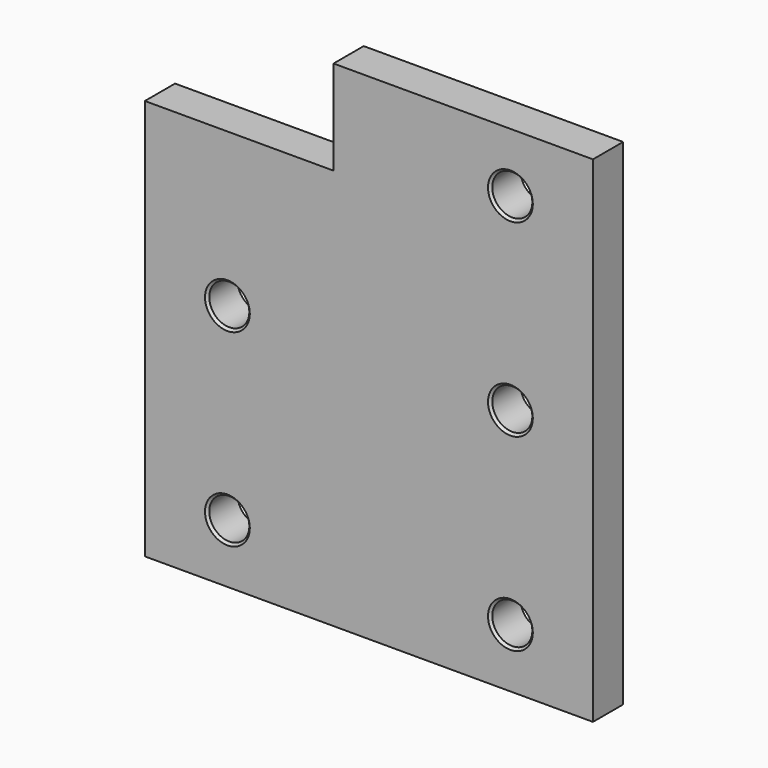
from build123d import *

# Parameters (mm, degrees)
F0_W     = 95
F0_H     = 105
F0_R     = 4.25
F1_DEPTH = 8
F2_SIZE  = 0.5
F3_W     = 50
F3_H     = 55.8646805584
F4_DEPTH = 25


with BuildPart() as f1:
    # F0 (on Front) → F1 (new body)
    with BuildSketch(Plane.XZ):
        with Locations((2.5, 0)):
            Rectangle(F0_W, F0_H)
        with Locations((-27.5, -40)):
            Circle(F0_R, mode=Mode.SUBTRACT)
        with Locations((32.5, -40)):
            Circle(F0_R, mode=Mode.SUBTRACT)
        with Locations((-27.5, 0)):
            Circle(F0_R, mode=Mode.SUBTRACT)
        with Locations((32.5, 0)):
            Circle(F0_R, mode=Mode.SUBTRACT)
        with Locations((32.5, 40)):
            Circle(F0_R, mode=Mode.SUBTRACT)
    extrude(amount=F1_DEPTH)

    # F2
    f2_edges = [f1.edges().sort_by_distance(p)[0] for p in [
        (28.25, -8, 40),
        (28.25, -8, -40),
        (-31.75, -8, -40),
        (-31.75, -8, 0),
        (28.25, -8, 0),
    ]]
    chamfer(f2_edges, length=F2_SIZE)

    # F3 (on face) → F4 (cut)
    with BuildSketch(Plane.XZ.offset(8)):
        with Locations((-30, 60.4323402792)):
            Rectangle(F3_W, F3_H)
    extrude(amount=-F4_DEPTH, mode=Mode.SUBTRACT)


solid = f1.part
